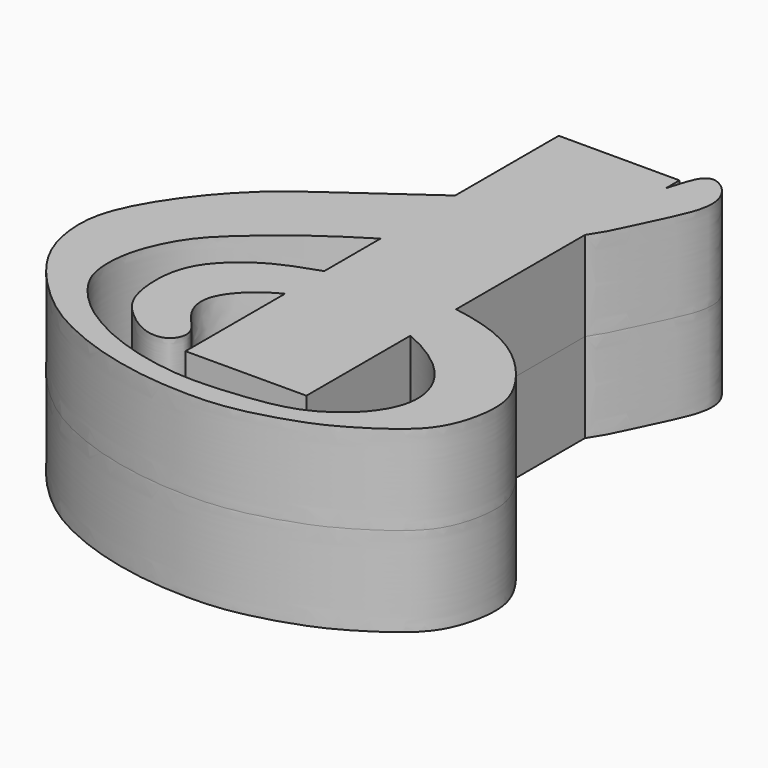
from build123d import *

# Parameters (mm, degrees)
F1_DEPTH  = 50.8
F3_DEPTH  = 50.8
F5_DEPTH  = 44.45
F8_DEPTH  = 6.35
F10_DEPTH = 6.35


with BuildPart() as f1:
    # F0 (on Top) → F1 (new body)
    with BuildSketch(Plane.XY):
        with BuildLine():
            add(Edge.make_bspline(
                [(39.2988994718, 181.5888132131), (34.1337236264, 179.8397306976), (30.792050612, 160.7818887429), (23.9946611028, 150.8584451747), (16.8897895888, 141.0112474832), (5.6229946118, 130.7380510814), (-1.5865514667, 124.8713086502), (-15.2454228269, 114.0871058767), (-32.5142332038, 102.6686575853), (-46.4053457188, 93.0851621285), (-82.8875423179, 66.7177850311), (-103.7650157797, 52.5784029052), (-127.2729420588, 28.9054443459), (-145.6947221807, 0.8150535386), (-153.292357857, -21.8780215764), (-150.0442937073, -47.5620358537), (-139.4345420152, -67.3345168154), (-123.4614337375, -84.9870981503), (-107.9510580384, -97.9527447323), (-91.973363835, -107.1533821065), (-70.8431634458, -115.889743821), (-49.4751207324, -121.1921073629), (-33.4799127178, -123.5956363048), (-17.9632238664, -124.7076173771), (10.0382100706, -125.0474077654), (46.2812714574, -113.8685036206), (61.8927456346, -105.7300693022), (79.0232630113, -95.205939733), (97.8509229946, -79.3025584959), (104.0306941137, -50.679616718), (100.2261318438, -32.846425904), (84.0797927563, -10.2610543395), (57.9009267675, 9.0144135813), (12.2429307109, 17.0083896833), (-17.444326242, 12.0621487333), (-54.1001364708, 1.0401296743), (-74.1550562144, -10.551036753), (-92.2816513275, -30.2229546496), (-92.0278464553, -58.620251525), (-86.5092490186, -72.4052036519), (-77.4696924273, -81.662744917), (-64.6520900375, -90.3490454216), (-50.8526379184, -89.8187261689), (-45.8695219514, -76.6293365535), (-59.8535306691, -65.3243801929), (-65.7829738943, -48.4970641146), (-53.9989284234, -31.0877996042), (-34.3114758802, -19.0740058075), (-11.574408223, -14.5449757252), (12.0109969689, -13.6595300471), (33.4946888487, -19.1318257627), (63.1838857193, -37.9052360967), (72.8098387023, -63.6839402312), (65.502661316, -82.8592074003), (52.7052199191, -96.1082515386), (34.4666663956, -107.2369447788), (8.2130377329, -111.2883782733), (-19.4367855334, -113.4035548404), (-40.9505241028, -111.0040217479), (-61.9784891794, -105.8416137592), (-82.2590981119, -97.2792515452), (-100.7536395892, -84.9813934063), (-115.0629752237, -68.0797874346), (-119.1069297291, -53.3437360072), (-117.8741715891, -32.6775535579), (-106.7993990184, -8.6741021072), (-89.8991678615, 8.4018360053), (-62.2015956638, 30.9805619458), (-32.0342228498, 49.4801478888), (-5.7756484913, 65.3192863422), (11.0358045177, 80.3465300933), (34.70941482, 109.0552885923), (43.9242233638, 133.5484779664), (63.0443465713, 167.8077860543), (44.2879751225, 183.2782629533), (39.2988994718, 181.5888132131)],
                knots=[0, 0, 0, 0, 0.0132998091, 0.0237205654, 0.033613614, 0.0446792372, 0.053494589, 0.0653830276, 0.0782970729, 0.0903873346, 0.1093828994, 0.1242388904, 0.1405948495, 0.1572512577, 0.1711473961, 0.1853931231, 0.198976292, 0.2129289953, 0.2257688659, 0.2380193525, 0.2517737824, 0.2653047639, 0.2766844378, 0.2877772103, 0.3030722055, 0.3207261277, 0.3327908843, 0.3453982054, 0.3595674756, 0.3746348965, 0.3867422055, 0.4014116972, 0.4178430285, 0.4369994727, 0.4530651046, 0.4705348861, 0.4844107014, 0.4987909845, 0.5136937812, 0.5245734407, 0.5347286727, 0.5459821449, 0.5558579603, 0.5650416704, 0.576724484, 0.5882869665, 0.6008095228, 0.6145331019, 0.6283511975, 0.642084502, 0.6556118497, 0.672374532, 0.6868640689, 0.6993348405, 0.7114937447, 0.7245627468, 0.7393716343, 0.7545226953, 0.7678406525, 0.7810951291, 0.794524117, 0.8081261841, 0.8213971051, 0.83238596, 0.8452526293, 0.8598048045, 0.8738691841, 0.8909564264, 0.9083009462, 0.9239311596, 0.9376755908, 0.9547726535, 0.9701053144, 0.9871536312, 1, 1, 1, 1], degree=3))
        make_face()
    extrude(amount=F1_DEPTH)

    # F2 (on face) → F3 (join)
    with BuildSketch(Plane.XY.offset(50.8)):
        with BuildLine():
            Line((-38.6916001286, 171.8740314245), (-38.6916001286, 98.3816893637))
            add(Edge.make_bspline(
                [(29.8883998714, 162.138891369), (28.071337649, 156.8099509586), (23.977193995, 150.8342361424), (16.8897895888, 141.0112474832), (5.6229946118, 130.7380510814), (-1.5865514667, 124.8713086502), (-15.2454228269, 114.0871058767), (-29.6936188335, 104.5336985831), (-36.3821621253, 99.9806712032), (-38.6916001286, 98.3816893637)],
                knots=[0.0133769545, 0.0133769545, 0.0133769545, 0.0133769545, 0.0237205654, 0.033613614, 0.0446792372, 0.053494589, 0.0653830276, 0.0782970729, 0.0843614298, 0.0843614298, 0.0843614298, 0.0843614298], degree=3))
            Line((29.8883998714, 162.138891369), (29.8883998714, 171.8740314245))
            Line((29.8883998714, 171.8740314245), (-38.6916001286, 171.8740314245))
        make_face()
        with BuildLine():
            add(Edge.make_bspline(
                [(29.8883998713, 13.2854365114), (23.9808988631, 14.2085358001), (5.6663622394, 15.9126571831), (-13.1273783483, 12.7814022664), (-31.891357926, 7.58583182), (-38.6916001286, 5.4058012194)],
                knots=[0.4295157677, 0.4295157677, 0.4295157677, 0.4295157677, 0.4369994727, 0.4530651046, 0.4628727432, 0.4628727432, 0.4628727432, 0.4628727432], degree=3))
            Line((29.8883998714, 13.2854365114), (29.8883998714, 104.708188787))
            add(Edge.make_bspline(
                [(-38.6916001286, 45.3611012718), (-36.236051587, 46.8737556834), (-24.6274259059, 53.9479183278), (-5.7756484913, 65.3192863422), (10.1146884782, 79.5231726333), (24.2691320278, 96.4187035869), (29.8883998714, 104.708188787)],
                knots=[0.9041345738, 0.9041345738, 0.9041345738, 0.9041345738, 0.9083009462, 0.9239311596, 0.9376755908, 0.9522264229, 0.9522264229, 0.9522264229, 0.9522264229], degree=3))
            Line((-38.6916001286, 45.3611012718), (-38.6916001286, 5.4058012194))
        make_face()
        with BuildLine():
            Line((22.5164723147, -12.8357740365), (29.8883998714, -12.8357740365))
            Line((29.8883998714, -12.8357740365), (29.8883998714, 13.2854365114))
            add(Edge.make_bspline(
                [(29.8883998713, 13.2854365114), (23.9808988631, 14.2085358001), (5.6663622394, 15.9126571831), (-13.1273783483, 12.7814022664), (-31.891357926, 7.58583182), (-38.6916001286, 5.4058012194)],
                knots=[0.4295157677, 0.4295157677, 0.4295157677, 0.4295157677, 0.4369994727, 0.4530651046, 0.4628727432, 0.4628727432, 0.4628727432, 0.4628727432], degree=3))
            Line((-38.6916001286, 5.4058012194), (-38.6916001286, -12.8357740365))
            Line((-38.6916001286, -12.8357740365), (22.5164723147, -12.8357740365))
        make_face()
        with BuildLine():
            Line((29.8883998714, -19.1894176518), (29.8883998714, -12.8357740365))
            Line((29.8883998714, -12.8357740365), (22.5164723147, -12.8357740365))
            Line((22.5164723147, -12.8357740365), (-38.6916001286, -12.8357740365))
            Line((-38.6916001286, -12.8357740365), (-38.6916001286, -22.4914223356))
            add(Edge.make_bspline(
                [(-38.6916001285, -22.4914223356), (-37.1385870197, -21.7308209263), (-28.4473456686, -17.9059210511), (-11.574408223, -14.5449757252), (10.9496620364, -13.699374791), (23.4993958421, -16.6068723833), (29.8883998714, -19.1894176518)],
                knots=[0.6114547764, 0.6114547764, 0.6114547764, 0.6114547764, 0.6145331019, 0.6283511975, 0.642084502, 0.6537633205, 0.6537633205, 0.6537633205, 0.6537633205], degree=3))
        make_face()
        with BuildLine():
            Line((29.8883998714, -92.9508890234), (29.8883998714, -19.1894176518))
            add(Edge.make_bspline(
                [(-38.6916001285, -22.4914223356), (-37.1385870197, -21.7308209263), (-28.4473456686, -17.9059210511), (-11.574408223, -14.5449757252), (10.9496620364, -13.699374791), (23.4993958421, -16.6068723833), (29.8883998714, -19.1894176518)],
                knots=[0.6114547764, 0.6114547764, 0.6114547764, 0.6114547764, 0.6145331019, 0.6283511975, 0.642084502, 0.6537633205, 0.6537633205, 0.6537633205, 0.6537633205], degree=3))
            Line((-38.6916001286, -22.4914223356), (-38.6916001286, -93.0920700751))
            Line((-38.6916001286, -93.0920700751), (29.8883998714, -92.9508890234))
        make_face()
        with BuildLine():
            add(Edge.make_bspline(
                [(-38.6916001286, 45.3611012718), (-36.236051587, 46.8737556834), (-24.6274259059, 53.9479183278), (-5.7756484913, 65.3192863422), (10.1146884782, 79.5231726333), (24.2691320278, 96.4187035869), (29.8883998714, 104.708188787)],
                knots=[0.9041345738, 0.9041345738, 0.9041345738, 0.9041345738, 0.9083009462, 0.9239311596, 0.9376755908, 0.9522264229, 0.9522264229, 0.9522264229, 0.9522264229], degree=3))
            Line((29.8883998714, 104.708188787), (29.8883998714, 162.138891369))
            add(Edge.make_bspline(
                [(29.8883998714, 162.138891369), (28.071337649, 156.8099509586), (23.977193995, 150.8342361424), (16.8897895888, 141.0112474832), (5.6229946118, 130.7380510814), (-1.5865514667, 124.8713086502), (-15.2454228269, 114.0871058767), (-29.6936188335, 104.5336985831), (-36.3821621253, 99.9806712032), (-38.6916001286, 98.3816893637)],
                knots=[0.0133769545, 0.0133769545, 0.0133769545, 0.0133769545, 0.0237205654, 0.033613614, 0.0446792372, 0.053494589, 0.0653830276, 0.0782970729, 0.0843614298, 0.0843614298, 0.0843614298, 0.0843614298], degree=3))
            Line((-38.6916001286, 98.3816893637), (-38.6916001286, 45.3611012718))
        make_face()
    extrude(amount=-F3_DEPTH)

    # F4 (on face) → F5 (cut)
    with BuildSketch(Plane(origin=(0, 0, 0), x_dir=(1, 0, 0), z_dir=(0, 0, -1))):
        with BuildLine():
            Line((25.9675770915, 84.1259685755), (-34.9924229085, 84.1259685755))
            Line((-34.9924229085, 84.1259685755), (-34.9924229085, 20.8228369761))
            add(Edge.make_bspline(
                [(-34.9924229086, 20.8228369761), (-34.6463951579, 20.6796678948), (-27.1195831561, 17.6414420755), (-11.574408223, 14.5449757252), (9.5530299444, 13.7518072949), (21.0781088692, 16.0819052648), (25.9675770915, 17.7332438893)],
                knots=[0.6138650859, 0.6138650859, 0.6138650859, 0.6138650859, 0.6145331019, 0.6283511975, 0.642084502, 0.6513308036, 0.6513308036, 0.6513308036, 0.6513308036], degree=3))
            Line((25.9675770915, 17.7332438893), (25.9675770915, 84.1259685755))
        make_face()
        with BuildLine():
            add(Edge.make_bspline(
                [(-34.9924229086, 20.8228369761), (-34.6463951579, 20.6796678948), (-27.1195831561, 17.6414420755), (-11.574408223, 14.5449757252), (9.5530299444, 13.7518072949), (21.0781088692, 16.0819052648), (25.9675770915, 17.7332438893)],
                knots=[0.6138650859, 0.6138650859, 0.6138650859, 0.6138650859, 0.6145331019, 0.6283511975, 0.642084502, 0.6513308036, 0.6513308036, 0.6513308036, 0.6513308036], degree=3))
            Line((-34.9924229085, 20.8228369761), (-34.9924229085, -6.5620693045))
            add(Edge.make_bspline(
                [(25.9675770915, -13.8441670982), (21.4192929853, -14.4297047467), (4.729365923, -15.7565427412), (-12.1322084241, -12.9472091053), (-29.3488985717, -8.2823228306), (-34.9924229085, -6.5620693045)],
                knots=[0.4311788408, 0.4311788408, 0.4311788408, 0.4311788408, 0.4369994727, 0.4530651046, 0.461106418, 0.461106418, 0.461106418, 0.461106418], degree=3))
            Line((25.9675770915, -13.8441670982), (25.9675770915, 17.7332438893))
        make_face()
        with BuildLine():
            add(Edge.make_bspline(
                [(25.9675770915, -13.8441670982), (21.4192929853, -14.4297047467), (4.729365923, -15.7565427412), (-12.1322084241, -12.9472091053), (-29.3488985717, -8.2823228306), (-34.9924229085, -6.5620693045)],
                knots=[0.4311788408, 0.4311788408, 0.4311788408, 0.4311788408, 0.4369994727, 0.4530651046, 0.461106418, 0.461106418, 0.461106418, 0.461106418], degree=3))
            Line((-34.9924229085, -6.5620693045), (-34.9924229085, -47.629228625))
            add(Edge.make_bspline(
                [(-34.9924229085, -47.629228625), (-33.7807890169, -48.3691907666), (-23.4481647567, -54.6592471441), (-5.7756484913, -65.3192863422), (8.9566867631, -78.4880703118), (21.1166898904, -92.6950468487), (25.9675770914, -99.2054763079)],
                knots=[0.9062327112, 0.9062327112, 0.9062327112, 0.9062327112, 0.9083009462, 0.9239311596, 0.9376755908, 0.949025372, 0.949025372, 0.949025372, 0.949025372], degree=3))
            Line((25.9675770915, -99.2054763079), (25.9675770915, -13.8441670982))
        make_face()
        with BuildLine():
            add(Edge.make_bspline(
                [(-34.9924229085, -47.629228625), (-33.7807890169, -48.3691907666), (-23.4481647567, -54.6592471441), (-5.7756484913, -65.3192863422), (8.9566867631, -78.4880703118), (21.1166898904, -92.6950468487), (25.9675770914, -99.2054763079)],
                knots=[0.9062327112, 0.9062327112, 0.9062327112, 0.9062327112, 0.9083009462, 0.9239311596, 0.9376755908, 0.949025372, 0.949025372, 0.949025372, 0.949025372], degree=3))
            Line((-34.9924229085, -47.629228625), (-34.9924229085, -100.9212989797))
            add(Edge.make_bspline(
                [(25.9675770915, -153.8691883104), (25.2497602235, -152.730121205), (22.4294601067, -148.6891105703), (16.8897895888, -141.0112474832), (5.6229946118, -130.7380510814), (-1.5865514667, -124.8713086502), (-15.2454228269, -114.0871058767), (-28.141284488, -105.5601299972), (-33.9775635212, -101.6122401067), (-34.9924229085, -100.9212989797)],
                knots=[0.0202126874, 0.0202126874, 0.0202126874, 0.0202126874, 0.0237205654, 0.033613614, 0.0446792372, 0.053494589, 0.0653830276, 0.0782970729, 0.0810450533, 0.0810450533, 0.0810450533, 0.0810450533], degree=3))
            Line((25.9675770915, -153.8691883104), (25.9675770915, -99.2054763079))
        make_face()
        with BuildLine():
            add(Edge.make_bspline(
                [(25.9675770915, -153.8691883104), (25.2497602235, -152.730121205), (22.4294601067, -148.6891105703), (16.8897895888, -141.0112474832), (5.6229946118, -130.7380510814), (-1.5865514667, -124.8713086502), (-15.2454228269, -114.0871058767), (-28.141284488, -105.5601299972), (-33.9775635212, -101.6122401067), (-34.9924229085, -100.9212989797)],
                knots=[0.0202126874, 0.0202126874, 0.0202126874, 0.0202126874, 0.0237205654, 0.033613614, 0.0446792372, 0.053494589, 0.0653830276, 0.0782970729, 0.0810450533, 0.0810450533, 0.0810450533, 0.0810450533], degree=3))
            Line((-34.9924229085, -100.9212989797), (-34.9924229085, -171.8740314245))
            Line((-34.9924229085, -171.8740314245), (25.9675770915, -171.8740314245))
            Line((25.9675770915, -171.8740314245), (25.9675770915, -153.8691883104))
        make_face()
    extrude(amount=-F5_DEPTH, mode=Mode.SUBTRACT)


with BuildPart() as f6_1:
    # F6: instance of F1
    add(f1.part.mirror(Plane.XY))

    # F7 (on face) → F8 (join)
    with BuildSketch(Plane.YZ.offset(-34.9924229085)):
        Polygon((-84.1259685755, -25.4), (48.2660345733, -25.4), (171.8740314245, -25.4), (171.8740314245, -19.05), (48.2660345733, -19.05), (-84.1259685755, -19.05), align=None)
    extrude(amount=F8_DEPTH)

    # F9 (on face) → F10 (join)
    with BuildSketch(Plane(origin=(25.9675770915, 0, 0), x_dir=(0, -1, 0), z_dir=(-1, 0, 0))):
        Polygon((84.1259685755, -19.05), (-100.3284305334, -19.05), (-171.8740314245, -19.05), (-171.8740314245, -25.4), (-100.3284305334, -25.4), (84.1259685755, -25.4), align=None)
    extrude(amount=F10_DEPTH)


solid = Compound([f1.part, f6_1.part])
